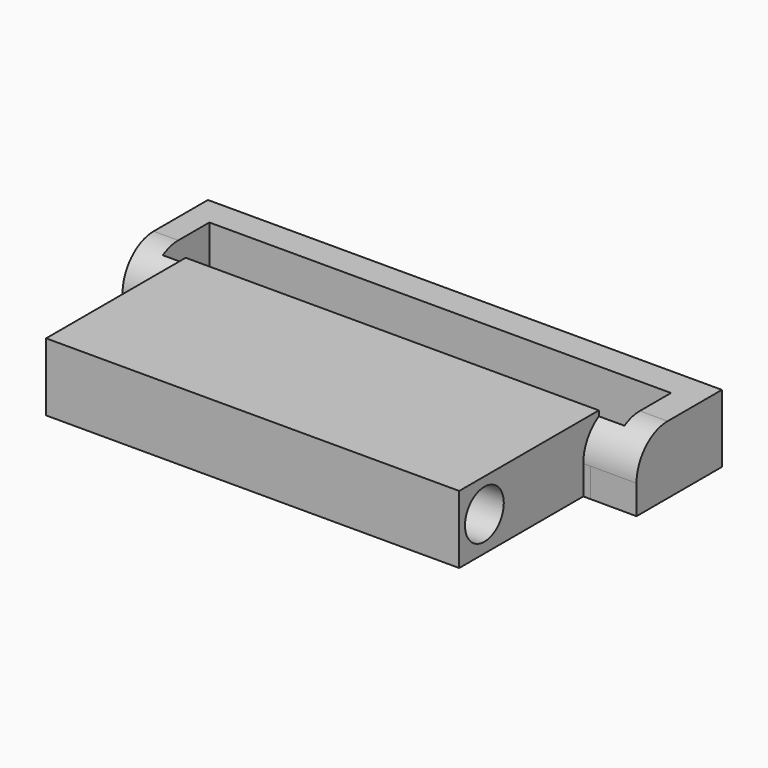
from build123d import *

# Parameters (mm, degrees)
F1_DEPTH      = 3.5
F2_R          = 1.25
F3_DEPTH      = 25
F3_DEPTH_BACK = 25
F4_T4_DEPTH   = 12.7513736877
F4_T9_DEPTH   = 12.4486649129


# Not quite as in the source:
# - a fillet or chamfer that OpenCascade refuses, or shapes differently, is made with other operations: its cross-section is extruded or revolved along the edge and cut away or added


with BuildPart() as f1:
    # F0 (on Top) → F1 (new body)
    with BuildSketch(Plane.XY):
        Polygon((-9.9924615563, -3.7976490931), (11.3075384437, -3.7976490931), (11.3075384437, 4.1987212708), (11.6869780256, 4.1973420195), (11.6869780256, 5.1973420195), (-10.3793237358, 5.1973420195), (-10.3752534696, 4.2007874551), (-9.9924615563, 4.2023509069), align=None)
        Polygon((11.6869780256, 5.1973420195), (11.6869780256, 4.1973420195), (14.0588939546, 4.1887201777), (14.0588939546, 9.6923498138), (-12.4411060454, 9.6923498138), (-12.4411060454, 4.1923498138), (-10.3752534696, 4.2007874551), (-10.3793237358, 5.1973420195), (-11.1709162593, 5.1973420195), (-11.1709162593, 8.1973420195), (12.6290837407, 8.1973420195), (12.6290837407, 5.1973420195), align=None)
    extrude(amount=F1_DEPTH)

    # F2 (on Right) → F3 (cut, two sides)
    with BuildSketch(Plane.YZ) as f3_sk:
        with Locations((-2.1757856011, 1.7836129991)):
            Circle(F2_R)
    extrude(amount=-F3_DEPTH, mode=Mode.SUBTRACT)
    extrude(f3_sk.sketch, amount=F3_DEPTH_BACK, mode=Mode.SUBTRACT)

    # F4: fillet of radius 2 on 2 edges, made by hand


with BuildPart() as f4_tool2:
    # F4_s3 → F4_t4 (new body)
    with BuildSketch(Plane(origin=(6.2921600495, -0.0228718094, 0), x_dir=(0, 0, 1), z_dir=(0.9999933936, -0.0036349454, 0))):
        with BuildLine():
            ThreePointArc((3.5, -6.2397958172), (2.9142135624, -4.8255822548), (1.5, -4.2397958172))
            Line((1.5, -4.2397958172), (3.5, -4.2397958172))
            Line((3.5, -4.2397958172), (3.5, -6.2397958172))
        make_face()
    extrude(amount=F4_T4_DEPTH)

    split(bisect_by=Plane.YZ.offset(11.3075384437), keep=Keep.TOP)


with BuildPart() as f1_1:
    add(f1.part)

    # F4_t1: cut F4_tool2
    add(f4_tool2.part, mode=Mode.SUBTRACT)


with BuildPart() as f4_tool7:
    # F4_s8 → F4_t9 (new body)
    with BuildSketch(Plane(origin=(-17.423734114, -0.0711644294, 0), x_dir=(0, 0, 1), z_dir=(0.9999916592, 0.0040843045, 0))):
        with BuildLine():
            ThreePointArc((3.5, -6.2431281117), (2.9142135624, -4.8289145493), (1.5, -4.2431281117))
            Line((1.5, -4.2431281117), (3.5, -4.2431281117))
            Line((3.5, -4.2431281117), (3.5, -6.2431281117))
        make_face()
    extrude(amount=F4_T9_DEPTH)

    split(bisect_by=Plane.YZ.offset(-9.9924615563), keep=Keep.BOTTOM)


with BuildPart() as f1_2:
    add(f1_1.part)

    # F4_t6: cut F4_tool7
    add(f4_tool7.part, mode=Mode.SUBTRACT)


solid = f1_2.part
